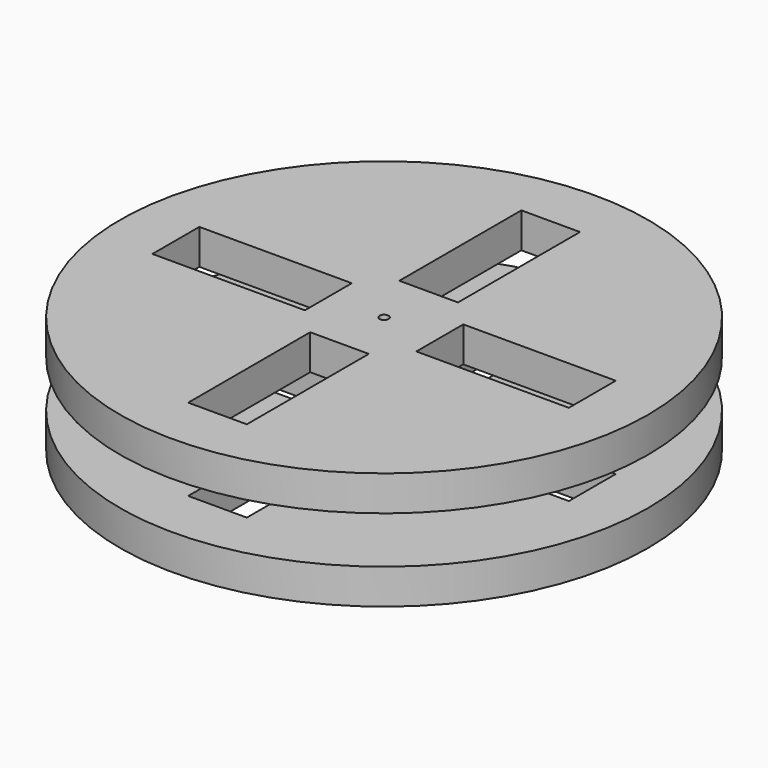
from build123d import *

# Parameters (mm, degrees)
F0_R     = 57.15
F0_R_2   = 0.9794958553
F1_DEPTH = 25.4
F3_T     = -7.62
F4_W     = 12.7
F4_H     = 33.02
F5_DEPTH = 25.4
F6_DEPTH = 25.4
F7_W     = 33.02
F7_H     = 6.35
F8_DEPTH = 25.4


# Not quite as in the source:
# - a feature of the source that left no trace in its solid (it failed there, or was rolled back) is left out


with BuildPart() as f1:
    # F0 (on Top) → F1 (new body)
    with BuildSketch(Plane.XY):
        Circle(F0_R)
        Circle(F0_R_2, mode=Mode.SUBTRACT)
    extrude(amount=F1_DEPTH)

    # F3
    f3_openings = [f1.faces().sort_by_distance(p)[0] for p in [
        (-57.15, 0, 12.7),
    ]]
    offset(amount=F3_T, openings=f3_openings)

    # F4 (on face) → F5 (cut)
    with BuildSketch(Plane.XY.offset(25.4)):
        with Locations((0, -28.575)):
            Rectangle(F4_W, F4_H)
    extrude(amount=-F5_DEPTH, mode=Mode.SUBTRACT)

    # F4 (on face) → F6 (cut)
    with BuildSketch(Plane.XY.offset(25.4)):
        with Locations((0, 28.575)):
            Rectangle(F4_W, F4_H)
        with Locations((0, -28.575)):
            Rectangle(F4_W, F4_H)
    extrude(amount=-F6_DEPTH, mode=Mode.SUBTRACT)

    # F7 (on face) → F8 (cut)
    with BuildSketch(Plane(origin=(0, 0, 0), x_dir=(1, 0, 0), z_dir=(0, 0, -1))):
        with Locations((28.575, 3.175)):
            Rectangle(F7_W, F7_H)
        with Locations((28.575, -3.175)):
            Rectangle(F7_W, F7_H)
        with Locations((-28.575, -3.175)):
            Rectangle(F7_W, F7_H)
        with Locations((-28.575, 3.175)):
            Rectangle(F7_W, F7_H)
    extrude(amount=-F8_DEPTH, mode=Mode.SUBTRACT)


solid = f1.part
